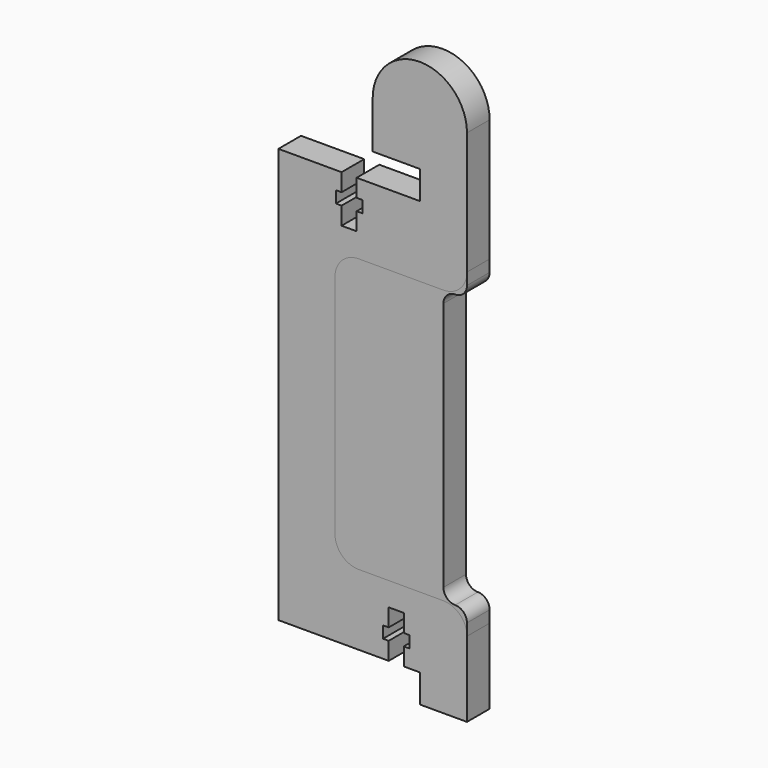
from build123d import *

# Parameters (mm, degrees)
F1_DEPTH  = 6
F3_DEPTH  = 6.001
F4_R      = 2
F5_DEPTH  = 6.001
F6_W      = 5
F6_H      = 58
F7_DEPTH  = 6.001
F8_R      = 2.49999
F10_DEPTH = 6
F11_DEPTH = 25
F12_W     = 28
F12_H     = 58
F13_DEPTH = 6
F14_R     = 5


# Not quite as in the source:
# - a fillet or chamfer is up to 0.001 mm smaller than in the source, because OpenCascade refuses the exact size


with BuildPart() as f1:
    # F0 (on Front) → F1 (new body)
    with BuildSketch(Plane.XZ):
        with BuildLine():
            Line((-10, 0), (0, 0))
            Line((0, 0), (0, 110))
            ThreePointArc((0, 110), (-10, 120), (-20, 110))
            Line((-20, 110), (-20, 100))
            Line((-20, 100), (-10, 100))
            Line((-10, 100), (-10, 94))
            Line((-10, 94), (-30, 94))
            Line((-30, 94), (-30, 6))
            Line((-30, 6), (-10, 6))
            Line((-10, 6), (-10, 0))
        make_face()
    extrude(amount=F1_DEPTH)

    # F2 (on face) → F3 (cut, through all)
    with BuildSketch(Plane.XZ.offset(6)):
        Polygon((-16.6, 6), (-15, 6), (-13.4, 6), (-13.4, 9.75), (-12.2, 9.75), (-12.2, 12.25), (-13.4, 12.25), (-13.4, 16), (-15, 16), (-16.6, 16), (-16.6, 12.25), (-17.8, 12.25), (-17.8, 9.75), (-16.6, 9.75), align=None)
        Polygon((-23.4, 94), (-25, 94), (-26.6, 94), (-26.6, 90.25), (-27.8, 90.25), (-27.8, 87.75), (-26.6, 87.75), (-26.6, 84), (-25, 84), (-23.4, 84), (-23.4, 87.75), (-22.2, 87.75), (-22.2, 90.25), (-23.4, 90.25), align=None)
    extrude(amount=-F3_DEPTH, mode=Mode.SUBTRACT)

    # F4 (on face) → F5 (cut, through all)
    with BuildSketch(Plane.XZ.offset(6)):
        with Locations((-10, 110)):
            Circle(F4_R)
    extrude(amount=-F5_DEPTH, mode=Mode.SUBTRACT)

    # F6 (on face) → F7 (cut, through all)
    with BuildSketch(Plane.XZ.offset(6)):
        with Locations((-2.5, 50)):
            Rectangle(F6_W, F6_H)
    extrude(amount=-F7_DEPTH, mode=Mode.SUBTRACT)

    # F8 (radius 2.5 in the source; OpenCascade refuses exactly that, so slightly less here)
    f8_edges = [f1.edges().sort_by_distance(p)[0] for p in [
        (-5, -3, 79),
        (0, -3, 79),
        (-5, -3, 21),
        (0, -3, 21),
    ]]
    fillet(f8_edges, radius=F8_R)


with BuildPart() as f10:
    # F9 (on Front) → F10 (new body)
    with BuildSketch(Plane.XZ):
        with BuildLine():
            Line((-10, 0), (0, 0))
            Line((0, 0), (0, 110))
            ThreePointArc((0, 110), (-10, 120), (-20, 110))
            Line((-20, 110), (-20, 100))
            Line((-20, 100), (-10, 100))
            Line((-10, 100), (-10, 94))
            Line((-10, 94), (-40, 94))
            Line((-40, 94), (-40, 6))
            Line((-40, 6), (-10, 6))
            Line((-10, 6), (-10, 0))
        make_face()
    extrude(amount=F10_DEPTH)

    # F2 (on face) → F11 (cut)
    with BuildSketch(Plane.XZ.offset(6)):
        Polygon((-16.6, 6), (-15, 6), (-13.4, 6), (-13.4, 9.75), (-12.2, 9.75), (-12.2, 12.25), (-13.4, 12.25), (-13.4, 16), (-15, 16), (-16.6, 16), (-16.6, 12.25), (-17.8, 12.25), (-17.8, 9.75), (-16.6, 9.75), align=None)
        Polygon((-23.4, 94), (-25, 94), (-26.6, 94), (-26.6, 90.25), (-27.8, 90.25), (-27.8, 87.75), (-26.6, 87.75), (-26.6, 84), (-25, 84), (-23.4, 84), (-23.4, 87.75), (-22.2, 87.75), (-22.2, 90.25), (-23.4, 90.25), align=None)
    extrude(amount=-F11_DEPTH, mode=Mode.SUBTRACT)

    # F12 (on Front) → F13 (cut, through all)
    with BuildSketch(Plane.XZ):
        with Locations((-14, 50)):
            Rectangle(F12_W, F12_H)
    extrude(amount=F13_DEPTH, mode=Mode.SUBTRACT)

    # F14
    f14_edges = [f10.edges().sort_by_distance(p)[0] for p in [
        (0, -3, 79),
        (0, -3, 21),
        (-28, -3, 21),
        (-28, -3, 79),
    ]]
    fillet(f14_edges, radius=F14_R)


solid = Compound([f1.part, f10.part])
